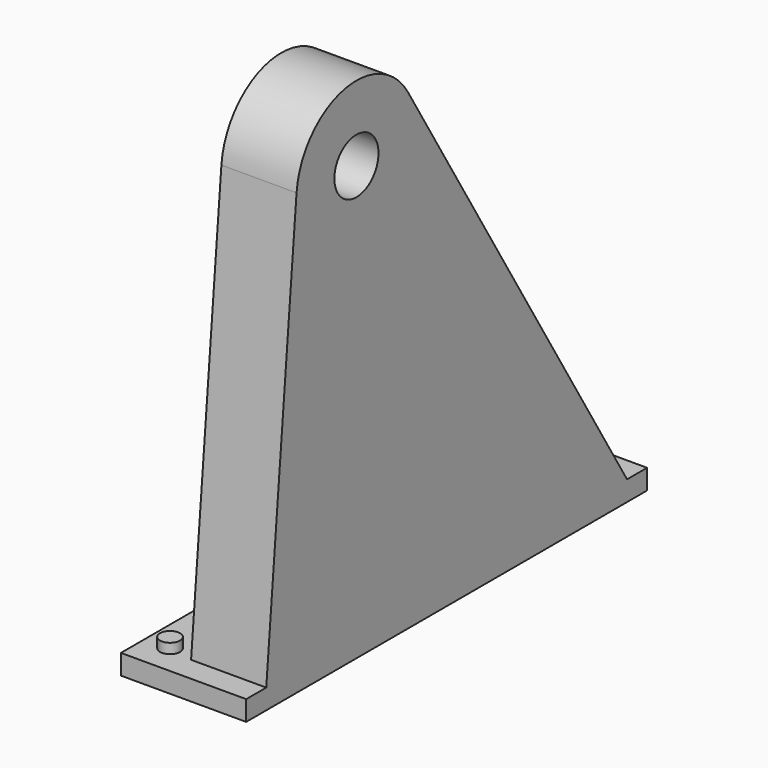
from build123d import *

# Parameters (mm, degrees)
F0_W          = 20
F0_H          = 0.8
F1_DEPTH      = 3
F1_DEPTH_BACK = 2
F2_R          = 1.1
F3_DEPTH      = 3
F5_DEPTH      = 1.5
F6_R          = 2
F7_R          = 1.49999
F8_R          = 0.4
F9_DEPTH      = 0.4


# Not quite as in the source:
# - a fillet or chamfer is up to 0.001 mm smaller than in the source, because OpenCascade refuses the exact size


with BuildPart() as f1:
    # F0 (on Right) → F1 (new body, two sides)
    with BuildSketch(Plane.YZ) as f1_sk:
        with Locations((4.5, 0.4)):
            Rectangle(F0_W, F0_H)
    extrude(amount=F1_DEPTH)
    extrude(f1_sk.sketch, amount=-F1_DEPTH_BACK)

    # F2 (on Right) → F3 (join)
    with BuildSketch(Plane.YZ):
        with BuildLine():
            Line((-4.5, 0.8), (13.5, 0.8))
            Line((13.5, 0.8), (2.5660948526, 18.8540776067))
            ThreePointArc((2.5660948526, 18.8540776067), (-0.6760626552, 20.2228306975), (-2.9878775484, 17.5694211496))
            Line((-2.9878775484, 17.5694211496), (-4.5, 0.8))
        make_face()
        with Locations((0, 17.3)):
            Circle(F2_R, mode=Mode.SUBTRACT)
    extrude(amount=F3_DEPTH)

    # F4 (on face) → F5 (cut)
    with BuildSketch(Plane(origin=(0, 0, 0), x_dir=(0, -1, 0), z_dir=(-1, 0, 0))):
        Polygon((-9.2406928099, 3.2), (1.8738512935, 3.2), (0.8819657168, 14.2), (-2.5788760591, 14.2), align=None)
    extrude(amount=-F5_DEPTH, mode=Mode.SUBTRACT)

    # F6
    f6_edges = [f1.edges().sort_by_distance(p)[0] for p in [
        (0.75, -0.881966, 14.2),
        (0.75, 2.578876, 14.2),
        (0.75, 9.240693, 3.2),
        (0.75, -1.873851, 3.2),
    ]]
    fillet(f6_edges, radius=F6_R)

    # F7 (radius 1.5 in the source; OpenCascade refuses exactly that, so slightly less here)
    f7_edges = [f1.edges().sort_by_distance(p)[0] for p in [
        (1.5, 3.002938, 3.2),
        (1.5, 7.433697, 4.218191),
        (1.5, -1.161746, 3.850783),
        (1.5, 5.282331, 9.736052),
        (1.5, -1.361712, 8.879614),
        (1.5, 2.433741, 13.942427),
        (1.5, -0.403411, 13.676352),
        (1.5, 1.198869, 14.2),
    ]]
    fillet(f7_edges, radius=F7_R)

    # F8 (on face) → F9 (join)
    with BuildSketch(Plane.XY.offset(0.8)):
        with Locations((-1, -4.3)):
            Circle(F8_R)
        with Locations((-1, -0.8)):
            Circle(F8_R)
        with Locations((-1, 2.7)):
            Circle(F8_R)
        with Locations((-1, 6.2)):
            Circle(F8_R)
        with Locations((-1, 9.7)):
            Circle(F8_R)
        with Locations((-1, 13.2)):
            Circle(F8_R)
    extrude(amount=F9_DEPTH)


solid = f1.part
